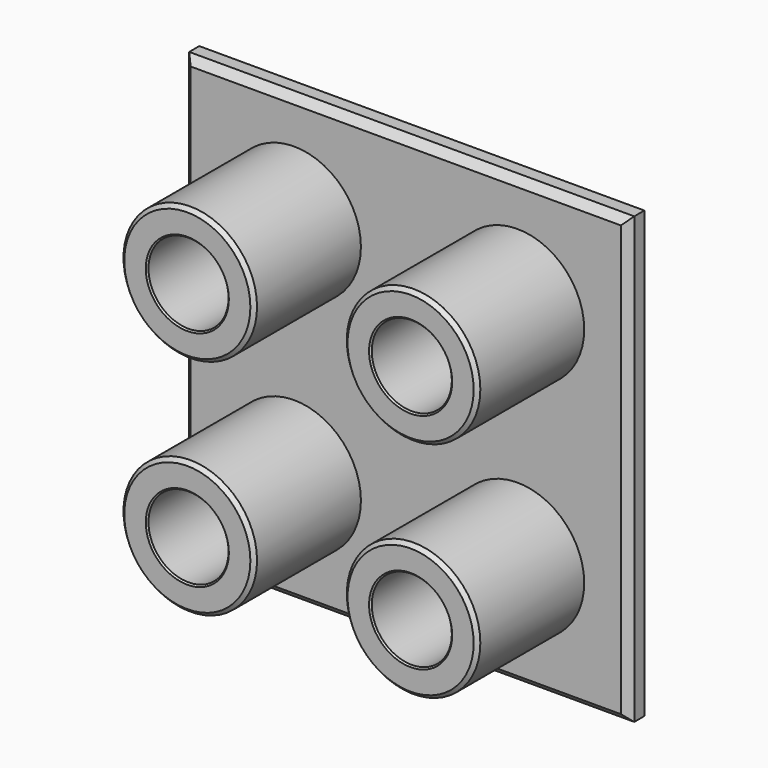
from build123d import *

# Parameters (mm, degrees)
F0_W         = 76.2
F0_H         = 76.2
F2_DEPTH     = 3.429
F1_R         = 4.2545
F3_DEPTH     = 3.556
F4_R         = 11.43
F4_R_2       = 6.858
F5_DEPTH     = 22.86
F6_SIZE      = 1.27
F7_SIZE      = 0.635
F8_SIZE      = 0.254
F9_TEXT_SIZE = 7.0555555556
F10_DEPTH    = 0.508


# Not quite as in the source:
# - Text() gives the source's letters only with a copy of the font that has no kerning and outlines rounded to 1/6400 em; it was checked with that copy


with BuildPart() as f2:
    # F0 (on Front) → F2 (new body)
    with BuildSketch(Plane.XZ):
        with Locations((-10.4464096949, 19.1454359185)):
            Rectangle(F0_W, F0_H)
    extrude(amount=F2_DEPTH)

    # F1 (on face) → F3 (cut)
    with BuildSketch(Plane.XZ):
        with Locations((-29.5599096949, 38.2589359185)):
            Circle(F1_R)
        with Locations((8.6670903051, 38.2589359185)):
            Circle(F1_R)
        with Locations((-29.5599096949, 0.0319359185)):
            Circle(F1_R)
        with Locations((8.6670903051, 0.0319359185)):
            Circle(F1_R)
    extrude(amount=F3_DEPTH, mode=Mode.SUBTRACT)

    # F4 (on face) → F5 (join)
    with BuildSketch(Plane.XZ.offset(3.429)):
        with Locations((-29.5599096949, 38.2589359185)):
            Circle(F4_R)
        with Locations((-29.5599096949, 38.2589359185)):
            Circle(F4_R_2, mode=Mode.SUBTRACT)
        with Locations((8.6670903051, 38.2589359185)):
            Circle(F4_R)
        with Locations((8.6670903051, 38.2589359185)):
            Circle(F4_R_2, mode=Mode.SUBTRACT)
        with Locations((-29.5599096949, 0.0319359185)):
            Circle(F4_R)
        with Locations((-29.5599096949, 0.0319359185)):
            Circle(F4_R_2, mode=Mode.SUBTRACT)
        with Locations((8.6670903051, 0.0319359185)):
            Circle(F4_R)
        with Locations((8.6670903051, 0.0319359185)):
            Circle(F4_R_2, mode=Mode.SUBTRACT)
    extrude(amount=F5_DEPTH)

    # F6
    f6_edges = [f2.edges().sort_by_distance(p)[0] for p in [
        (-10.44641, -3.429, 57.245436),
        (27.65359, -3.429, 19.145436),
        (-10.44641, -3.429, -18.954564),
        (-48.54641, -3.429, 19.145436),
    ]]
    chamfer(f6_edges, length=F6_SIZE)

    # F7
    f7_edges = [f2.edges().sort_by_distance(p)[0] for p in [
        (-40.98991, -26.289, 38.258936),
        (-2.76291, -26.289, 38.258936),
        (-2.76291, -26.289, 0.031936),
        (-40.98991, -26.289, 0.031936),
    ]]
    chamfer(f7_edges, length=F7_SIZE)

    # F8
    f8_edges = [f2.edges().sort_by_distance(p)[0] for p in [
        (-36.41791, -26.289, 38.258936),
        (1.80909, -26.289, 38.258936),
        (1.80909, -26.289, 0.031936),
        (-36.41791, -26.289, 0.031936),
    ]]
    chamfer(f8_edges, length=F8_SIZE)

    # F9 (on face) → F10 (join)
    with BuildSketch(Plane.XZ.offset(3.429)):
        with Locations((-16.302520806, 16.6054359185)):
            Text('R.L.', F9_TEXT_SIZE, font='Open Sans', text_align=(TextAlign.LEFT, TextAlign.BOTTOM))
    extrude(amount=F10_DEPTH)


solid = f2.part
